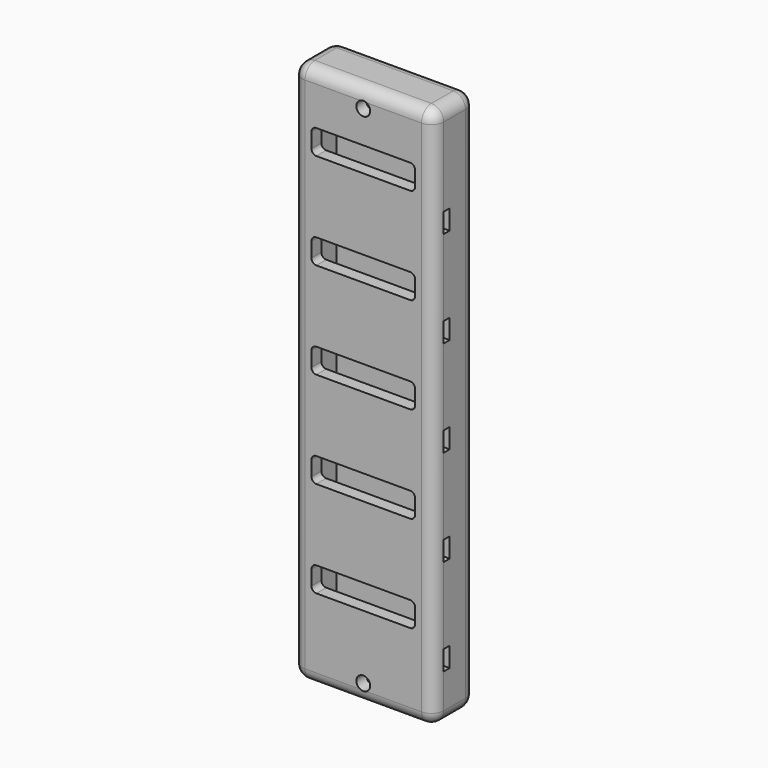
from build123d import *

# Parameters (mm, degrees)
F0_W         = 29.972
F0_H         = 5.08
F0_H_2       = 2.54
F0_R         = 1.7145
F0_H_3       = 13.97
F0_W_2       = 3.175
F1_DEPTH     = 10.16
F2_DEPTH     = 6.985
F3_DEPTH     = 1.905
F4_T1_DEPTH  = 133.35
F4_T3_DEPTH  = 14.9225
F4_T5_DEPTH  = 29.972
F4_S9_W      = 3.175
F4_S9_H      = 3.175
F4_T10_DEPTH = 3.175
F4_S15_W     = 3.175
F4_S15_H     = 3.175
F4_T16_DEPTH = 3.175
F4_S21_W     = 3.175
F4_S21_H     = 3.175
F4_T22_DEPTH = 3.175
F4_S27_W     = 3.175
F4_S27_H     = 3.175
F4_T28_DEPTH = 3.175
F5_R         = 1.778
F6_DEPTH     = 3.175
F7_T1_DEPTH  = 133.35
F7_T3_DEPTH  = 29.972
F7_T6_ANGLE  = 90
F7_T8_ANGLE  = 90
F7_T10_ANGLE = 90
F7_T12_ANGLE = 90


# Not quite as in the source:
# - a fillet or chamfer that OpenCascade refuses, or shapes differently, is made with other operations: its cross-section is extruded or revolved along the edge and cut away or added


with BuildPart() as f1:
    # F0 (on Front) → F1 (new body)
    with BuildSketch(Plane.XZ):
        with Locations((0, 14.605)):
            Rectangle(F0_W, F0_H)
        Polygon((-18.161, 86.36), (-18.161, 66.675), (-14.986, 66.675), (-14.986, 80.645), (14.986, 80.645), (14.986, 66.675), (18.161, 66.675), (18.161, 86.36), (14.986, 86.36), (14.986, 83.82), (-14.986, 83.82), (-14.986, 86.36), align=None)
        with Locations((0, 60.325)):
            Rectangle(F0_W, F0_H_2)
        Polygon((-18.161, 12.065), (-18.161, 0), (18.161, 0), (18.161, 12.065), (14.986, 12.065), (14.986, 9.525), (-14.986, 9.525), (-14.986, 12.065), align=None)
        with Locations((0, 4.7625)):
            Circle(F0_R, mode=Mode.SUBTRACT)
        with Locations((0, 85.09)):
            Rectangle(F0_W, F0_H_2)
        with Locations((0, 98.425)):
            Rectangle(F0_W, F0_H_3)
        Polygon((-18.161, 139.7), (-18.161, 116.205), (-14.986, 116.205), (-14.986, 130.175), (14.986, 130.175), (14.986, 116.205), (18.161, 116.205), (18.161, 139.7), align=None)
        with Locations((0, 134.9375)):
            Circle(F0_R, mode=Mode.SUBTRACT)
        with Locations((0, 48.895)):
            Rectangle(F0_W, F0_H_3)
        with Locations((0, 10.795)):
            Rectangle(F0_W, F0_H_2)
        with Locations((-16.5735, 39.37)):
            Rectangle(F0_W_2, F0_H)
        with Locations((0, 73.66)):
            Rectangle(F0_W, F0_H_3)
        with Locations((-16.5735, 14.605)):
            Rectangle(F0_W_2, F0_H)
        with Locations((0, 123.19)):
            Rectangle(F0_W, F0_H_3)
        with Locations((0, 109.855)):
            Rectangle(F0_W, F0_H_2)
        with Locations((0, 24.13)):
            Rectangle(F0_W, F0_H_3)
        with Locations((0, 35.56)):
            Rectangle(F0_W, F0_H_2)
        with Locations((-16.5735, 113.665)):
            Rectangle(F0_W_2, F0_H)
        with Locations((-16.5735, 64.135)):
            Rectangle(F0_W_2, F0_H)
        with Locations((0, 113.665)):
            Rectangle(F0_W, F0_H)
        Polygon((-18.161, 36.83), (-18.161, 17.145), (-14.986, 17.145), (-14.986, 31.115), (14.986, 31.115), (14.986, 17.145), (18.161, 17.145), (18.161, 36.83), (14.986, 36.83), (14.986, 34.29), (-14.986, 34.29), (-14.986, 36.83), align=None)
        with Locations((0, 39.37)):
            Rectangle(F0_W, F0_H)
        Polygon((-18.161, 111.125), (-18.161, 91.44), (-14.986, 91.44), (-14.986, 105.41), (14.986, 105.41), (14.986, 91.44), (18.161, 91.44), (18.161, 111.125), (14.986, 111.125), (14.986, 108.585), (-14.986, 108.585), (-14.986, 111.125), align=None)
        Polygon((-18.161, 61.595), (-18.161, 41.91), (-14.986, 41.91), (-14.986, 55.88), (14.986, 55.88), (14.986, 41.91), (18.161, 41.91), (18.161, 61.595), (14.986, 61.595), (14.986, 59.055), (-14.986, 59.055), (-14.986, 61.595), align=None)
        with Locations((0, 64.135)):
            Rectangle(F0_W, F0_H)
        with Locations((-16.5735, 88.9)):
            Rectangle(F0_W_2, F0_H)
        with Locations((0, 88.9)):
            Rectangle(F0_W, F0_H)
        with Locations((16.5735, 39.37)):
            Rectangle(F0_W_2, F0_H)
        with Locations((16.5735, 14.605)):
            Rectangle(F0_W_2, F0_H)
        with Locations((16.5735, 88.9)):
            Rectangle(F0_W_2, F0_H)
        with Locations((16.5735, 113.665)):
            Rectangle(F0_W_2, F0_H)
        with Locations((16.5735, 64.135)):
            Rectangle(F0_W_2, F0_H)
    extrude(amount=-F1_DEPTH)

    # F0 (on Front) → F2 (cut)
    with BuildSketch(Plane.XZ):
        with Locations((0, 98.425)):
            Rectangle(F0_W, F0_H_3)
        with Locations((0, 35.56)):
            Rectangle(F0_W, F0_H_2)
        with Locations((0, 48.895)):
            Rectangle(F0_W, F0_H_3)
        with Locations((0, 64.135)):
            Rectangle(F0_W, F0_H)
        with Locations((0, 14.605)):
            Rectangle(F0_W, F0_H)
        with Locations((0, 10.795)):
            Rectangle(F0_W, F0_H_2)
        with Locations((0, 113.665)):
            Rectangle(F0_W, F0_H)
        with Locations((0, 88.9)):
            Rectangle(F0_W, F0_H)
        with Locations((0, 123.19)):
            Rectangle(F0_W, F0_H_3)
        with Locations((0, 60.325)):
            Rectangle(F0_W, F0_H_2)
        with Locations((0, 24.13)):
            Rectangle(F0_W, F0_H_3)
        with Locations((0, 73.66)):
            Rectangle(F0_W, F0_H_3)
        with Locations((0, 39.37)):
            Rectangle(F0_W, F0_H)
        with Locations((0, 85.09)):
            Rectangle(F0_W, F0_H_2)
        with Locations((0, 109.855)):
            Rectangle(F0_W, F0_H_2)
    extrude(amount=-F2_DEPTH, mode=Mode.SUBTRACT)

    # F0 (on Front) → F3 (cut)
    with BuildSketch(Plane.XZ):
        with Locations((-16.5735, 14.605)):
            Rectangle(F0_W_2, F0_H)
        with Locations((0, 14.605)):
            Rectangle(F0_W, F0_H)
        with Locations((16.5735, 14.605)):
            Rectangle(F0_W_2, F0_H)
        with Locations((16.5735, 39.37)):
            Rectangle(F0_W_2, F0_H)
        with Locations((0, 39.37)):
            Rectangle(F0_W, F0_H)
        with Locations((-16.5735, 39.37)):
            Rectangle(F0_W_2, F0_H)
        with Locations((-16.5735, 88.9)):
            Rectangle(F0_W_2, F0_H)
        with Locations((0, 88.9)):
            Rectangle(F0_W, F0_H)
        with Locations((16.5735, 88.9)):
            Rectangle(F0_W_2, F0_H)
        with Locations((16.5735, 64.135)):
            Rectangle(F0_W_2, F0_H)
        with Locations((0, 64.135)):
            Rectangle(F0_W, F0_H)
        with Locations((-16.5735, 64.135)):
            Rectangle(F0_W_2, F0_H)
        with Locations((-16.5735, 113.665)):
            Rectangle(F0_W_2, F0_H)
        with Locations((0, 113.665)):
            Rectangle(F0_W, F0_H)
        with Locations((16.5735, 113.665)):
            Rectangle(F0_W_2, F0_H)
    extrude(amount=-F3_DEPTH, mode=Mode.SUBTRACT)

    # F4: fillet of radius 3.175 on 8 edges, made by hand

    # F4_s2 → F4_t1 (cut)
    with BuildSketch(Plane.XY.offset(3.175)):
        with BuildLine():
            ThreePointArc((18.161, 6.985), (17.2310640303, 9.2300640303), (14.986, 10.16))
            Line((14.986, 10.16), (18.161, 10.16))
            Line((18.161, 10.16), (18.161, 6.985))
        make_face()
        with BuildLine():
            ThreePointArc((-18.161, 6.985), (-17.2310640303, 9.2300640303), (-14.986, 10.16))
            Line((-14.986, 10.16), (-18.161, 10.16))
            Line((-18.161, 10.16), (-18.161, 6.985))
        make_face()
    extrude(amount=F4_T1_DEPTH, mode=Mode.SUBTRACT)

    # F4_s4 → F4_t3 (cut)
    with BuildSketch(Plane.XZ.offset(-6.985)):
        with BuildLine():
            ThreePointArc((18.161, 136.525), (17.2310640303, 138.7700640303), (14.986, 139.7))
            Line((14.986, 139.7), (18.161, 139.7))
            Line((18.161, 139.7), (18.161, 136.525))
        make_face()
        with BuildLine():
            ThreePointArc((-18.161, 136.525), (-17.2310640303, 138.7700640303), (-14.986, 139.7))
            Line((-14.986, 139.7), (-18.161, 139.7))
            Line((-18.161, 139.7), (-18.161, 136.525))
        make_face()
        with BuildLine():
            ThreePointArc((-14.986, 0), (-17.2310640303, 0.9299359697), (-18.161, 3.175))
            Line((-18.161, 3.175), (-18.161, 0))
            Line((-18.161, 0), (-14.986, 0))
        make_face()
        with BuildLine():
            ThreePointArc((14.986, 0), (17.2310640303, 0.9299359697), (18.161, 3.175))
            Line((18.161, 3.175), (18.161, 0))
            Line((18.161, 0), (14.986, 0))
        make_face()
    extrude(amount=F4_T3_DEPTH, mode=Mode.SUBTRACT)

    # F4_s6 → F4_t5 (cut)
    with BuildSketch(Plane.YZ.offset(-14.986)):
        with BuildLine():
            ThreePointArc((6.985, 0), (9.2300640303, 0.9299359697), (10.16, 3.175))
            Line((10.16, 3.175), (10.16, 0))
            Line((10.16, 0), (6.985, 0))
        make_face()
        with BuildLine():
            ThreePointArc((10.16, 136.525), (9.2300640303, 138.7700640303), (6.985, 139.7))
            Line((6.985, 139.7), (10.16, 139.7))
            Line((10.16, 139.7), (10.16, 136.525))
        make_face()
    extrude(amount=F4_T5_DEPTH, mode=Mode.SUBTRACT)


with BuildPart() as f4_tool8:
    # F4_s9 → F4_t10 (new body)
    with BuildSketch(Plane.XY.offset(3.175)):
        with Locations((16.5735, 8.5725)):
            Rectangle(F4_S9_W, F4_S9_H)
    extrude(amount=-F4_T10_DEPTH)

    # F4_s11 → F4_t12 (revolve, cut)
    with BuildSketch(Plane(origin=(14.986, 6.985, 3.175), x_dir=(-0.7071067812, -0.7071067812, 0), z_dir=(0.7071067812, -0.7071067812, 0))):
        with BuildLine():
            ThreePointArc((0, -3.175), (3.175, 0), (0, 3.175))
            Line((0, 3.175), (0, -3.175))
        make_face()
    revolve(axis=Axis((14.986, 6.985, 3.175), (0, 0, -1)), mode=Mode.SUBTRACT)


with BuildPart() as f1_1:
    add(f1.part)

    # F4_t7: cut F4_tool8
    add(f4_tool8.part, mode=Mode.SUBTRACT)


with BuildPart() as f4_tool14:
    # F4_s15 → F4_t16 (new body)
    with BuildSketch(Plane.XY.offset(136.525)):
        with Locations((16.5735, 8.5725)):
            Rectangle(F4_S15_W, F4_S15_H)
    extrude(amount=F4_T16_DEPTH)

    # F4_s17 → F4_t18 (revolve, cut)
    with BuildSketch(Plane(origin=(14.986, 6.985, 136.525), x_dir=(-0.7071067812, -0.7071067812, 0), z_dir=(-0.7071067812, 0.7071067812, 0))):
        with BuildLine():
            ThreePointArc((0, -3.175), (3.175, 0), (0, 3.175))
            Line((0, 3.175), (0, -3.175))
        make_face()
    revolve(axis=Axis((14.986, 6.985, 136.525), (0, 0, 1)), mode=Mode.SUBTRACT)


with BuildPart() as f1_2:
    add(f1_1.part)

    # F4_t13: cut F4_tool14
    add(f4_tool14.part, mode=Mode.SUBTRACT)


with BuildPart() as f4_tool20:
    # F4_s21 → F4_t22 (new body)
    with BuildSketch(Plane.YZ.offset(-14.986)):
        with Locations((8.5725, 138.1125)):
            Rectangle(F4_S21_W, F4_S21_H)
    extrude(amount=-F4_T22_DEPTH)

    # F4_s23 → F4_t24 (revolve, cut)
    with BuildSketch(Plane(origin=(-14.986, 6.985, 136.525), x_dir=(0, -0.7071067812, -0.7071067812), z_dir=(0, 0.7071067812, -0.7071067812))):
        with BuildLine():
            ThreePointArc((0, -3.175), (3.175, 0), (0, 3.175))
            Line((0, 3.175), (0, -3.175))
        make_face()
    revolve(axis=Axis((-14.986, 6.985, 136.525), (-1, 0, 0)), mode=Mode.SUBTRACT)


with BuildPart() as f1_3:
    add(f1_2.part)

    # F4_t19: cut F4_tool20
    add(f4_tool20.part, mode=Mode.SUBTRACT)


with BuildPart() as f4_tool26:
    # F4_s27 → F4_t28 (new body)
    with BuildSketch(Plane.XY.offset(3.175)):
        with Locations((-16.5735, 8.5725)):
            Rectangle(F4_S27_W, F4_S27_H)
    extrude(amount=-F4_T28_DEPTH)

    # F4_s29 → F4_t30 (revolve, cut)
    with BuildSketch(Plane(origin=(-14.986, 6.985, 3.175), x_dir=(0.7071067812, -0.7071067812, 0), z_dir=(0.7071067812, 0.7071067812, 0))):
        with BuildLine():
            ThreePointArc((0, -3.175), (3.175, 0), (0, 3.175))
            Line((0, 3.175), (0, -3.175))
        make_face()
    revolve(axis=Axis((-14.986, 6.985, 3.175), (0, 0, -1)), mode=Mode.SUBTRACT)


with BuildPart() as f1_4:
    add(f1_3.part)

    # F4_t25: cut F4_tool26
    add(f4_tool26.part, mode=Mode.SUBTRACT)


with BuildPart() as f6:
    # F5 (on Front) → F6 (new body)
    with BuildSketch(Plane.XZ):
        with BuildLine():
            ThreePointArc((-18.161, 3.175), (-17.2310640303, 0.9299359697), (-14.986, 0))
            Line((-14.986, 0), (14.986, 0))
            ThreePointArc((14.986, 0), (17.2310640303, 0.9299359697), (18.161, 3.175))
            Line((18.161, 3.175), (18.161, 136.525))
            ThreePointArc((18.161, 136.525), (17.2310640303, 138.7700640303), (14.986, 139.7))
            Line((14.986, 139.7), (-14.986, 139.7))
            ThreePointArc((-14.986, 139.7), (-17.2310640303, 138.7700640303), (-18.161, 136.525))
            Line((-18.161, 136.525), (-18.161, 3.175))
        make_face()
        with Locations((0, 4.7625)):
            Circle(F5_R, mode=Mode.SUBTRACT)
        with BuildLine():
            Line((12.065, 21.209), (-12.065, 21.209))
            ThreePointArc((-12.065, 21.209), (-12.9630256121, 21.5809743879), (-13.335, 22.479))
            Line((-13.335, 22.479), (-13.335, 26.289))
            ThreePointArc((-13.335, 26.289), (-12.9630256121, 27.1870256121), (-12.065, 27.559))
            Line((-12.065, 27.559), (12.065, 27.559))
            ThreePointArc((12.065, 27.559), (12.9630256121, 27.1870256121), (13.335, 26.289))
            Line((13.335, 26.289), (13.335, 22.479))
            ThreePointArc((13.335, 22.479), (12.9630256121, 21.5809743879), (12.065, 21.209))
        make_face(mode=Mode.SUBTRACT)
        with BuildLine():
            Line((12.065, 45.974), (-12.065, 45.974))
            ThreePointArc((-12.065, 45.974), (-12.9630256121, 46.3459743879), (-13.335, 47.244))
            Line((-13.335, 47.244), (-13.335, 51.054))
            ThreePointArc((-13.335, 51.054), (-12.9630256121, 51.9520256121), (-12.065, 52.324))
            Line((-12.065, 52.324), (12.065, 52.324))
            ThreePointArc((12.065, 52.324), (12.9630256121, 51.9520256121), (13.335, 51.054))
            Line((13.335, 51.054), (13.335, 47.244))
            ThreePointArc((13.335, 47.244), (12.9630256121, 46.3459743879), (12.065, 45.974))
        make_face(mode=Mode.SUBTRACT)
        with BuildLine():
            Line((12.065, 70.739), (-12.065, 70.739))
            ThreePointArc((-12.065, 70.739), (-12.9630256121, 71.1109743879), (-13.335, 72.009))
            Line((-13.335, 72.009), (-13.335, 75.819))
            ThreePointArc((-13.335, 75.819), (-12.9630256121, 76.7170256121), (-12.065, 77.089))
            Line((-12.065, 77.089), (12.065, 77.089))
            ThreePointArc((12.065, 77.089), (12.9630256121, 76.7170256121), (13.335, 75.819))
            Line((13.335, 75.819), (13.335, 72.009))
            ThreePointArc((13.335, 72.009), (12.9630256121, 71.1109743879), (12.065, 70.739))
        make_face(mode=Mode.SUBTRACT)
        with BuildLine():
            Line((12.065, 95.504), (-12.065, 95.504))
            ThreePointArc((-12.065, 95.504), (-12.9630256121, 95.8759743879), (-13.335, 96.774))
            Line((-13.335, 96.774), (-13.335, 100.584))
            ThreePointArc((-13.335, 100.584), (-12.9630256121, 101.4820256121), (-12.065, 101.854))
            Line((-12.065, 101.854), (12.065, 101.854))
            ThreePointArc((12.065, 101.854), (12.9630256121, 101.4820256121), (13.335, 100.584))
            Line((13.335, 100.584), (13.335, 96.774))
            ThreePointArc((13.335, 96.774), (12.9630256121, 95.8759743879), (12.065, 95.504))
        make_face(mode=Mode.SUBTRACT)
        with BuildLine():
            Line((12.065, 120.269), (-12.065, 120.269))
            ThreePointArc((-12.065, 120.269), (-12.9630256121, 120.6409743879), (-13.335, 121.539))
            Line((-13.335, 121.539), (-13.335, 125.349))
            ThreePointArc((-13.335, 125.349), (-12.9630256121, 126.2470256121), (-12.065, 126.619))
            Line((-12.065, 126.619), (12.065, 126.619))
            ThreePointArc((12.065, 126.619), (12.9630256121, 126.2470256121), (13.335, 125.349))
            Line((13.335, 125.349), (13.335, 121.539))
            ThreePointArc((13.335, 121.539), (12.9630256121, 120.6409743879), (12.065, 120.269))
        make_face(mode=Mode.SUBTRACT)
        with Locations((0, 134.9375)):
            Circle(F5_R, mode=Mode.SUBTRACT)
    extrude(amount=F6_DEPTH)

    # F7: fillet of radius 3.175 on 8 edges, made by hand

    # F7_s2 → F7_t1 (cut)
    with BuildSketch(Plane.XY.offset(3.175)):
        with BuildLine():
            ThreePointArc((18.161, 0), (17.2310640303, -2.2450640303), (14.986, -3.175))
            Line((14.986, -3.175), (18.161, -3.175))
            Line((18.161, -3.175), (18.161, 0))
        make_face()
        with BuildLine():
            ThreePointArc((-18.161, 0), (-17.2310640303, -2.2450640303), (-14.986, -3.175))
            Line((-14.986, -3.175), (-18.161, -3.175))
            Line((-18.161, -3.175), (-18.161, 0))
        make_face()
    extrude(amount=F7_T1_DEPTH, mode=Mode.SUBTRACT)

    # F7_s4 → F7_t3 (cut)
    with BuildSketch(Plane.YZ.offset(-14.986)):
        with BuildLine():
            ThreePointArc((0, 0), (-2.2450640303, 0.9299359697), (-3.175, 3.175))
            Line((-3.175, 3.175), (-3.175, 0))
            Line((-3.175, 0), (0, 0))
        make_face()
        with BuildLine():
            ThreePointArc((0, 139.7), (-2.2450640303, 138.7700640303), (-3.175, 136.525))
            Line((-3.175, 136.525), (-3.175, 139.7))
            Line((-3.175, 139.7), (0, 139.7))
        make_face()
    extrude(amount=F7_T3_DEPTH, mode=Mode.SUBTRACT)

    # F7_s5 → F7_t6 (revolve, cut)
    with BuildSketch(Plane.XY.offset(3.175)):
        with BuildLine():
            ThreePointArc((-18.161, 0), (-17.2310640303, -2.2450640303), (-14.986, -3.175))
            Line((-14.986, -3.175), (-18.161, -3.175))
            Line((-18.161, -3.175), (-18.161, 0))
        make_face()
    revolve(axis=Axis((-14.986, -3.175, 3.175), (0, -1, 0)), revolution_arc=F7_T6_ANGLE, mode=Mode.SUBTRACT)

    # F7_s7 → F7_t8 (revolve, cut)
    with BuildSketch(Plane.YZ.offset(14.986)):
        with BuildLine():
            ThreePointArc((0, 0), (-2.2450640303, 0.9299359697), (-3.175, 3.175))
            Line((-3.175, 3.175), (-3.175, 0))
            Line((-3.175, 0), (0, 0))
        make_face()
    revolve(axis=Axis((14.986, -3.175, 3.175), (0, -1, 0)), revolution_arc=F7_T8_ANGLE, mode=Mode.SUBTRACT)

    # F7_s9 → F7_t10 (revolve, cut)
    with BuildSketch(Plane.XY.offset(136.525)):
        with BuildLine():
            ThreePointArc((18.161, 0), (17.2310640303, -2.2450640303), (14.986, -3.175))
            Line((14.986, -3.175), (18.161, -3.175))
            Line((18.161, -3.175), (18.161, 0))
        make_face()
    revolve(axis=Axis((14.986, -3.175, 136.525), (0, -1, 0)), revolution_arc=F7_T10_ANGLE, mode=Mode.SUBTRACT)

    # F7_s11 → F7_t12 (revolve, cut)
    with BuildSketch(Plane.YZ.offset(-14.986)):
        with BuildLine():
            ThreePointArc((0, 139.7), (-2.2450640303, 138.7700640303), (-3.175, 136.525))
            Line((-3.175, 136.525), (-3.175, 139.7))
            Line((-3.175, 139.7), (0, 139.7))
        make_face()
    revolve(axis=Axis((-14.986, -3.175, 136.525), (0, -1, 0)), revolution_arc=F7_T12_ANGLE, mode=Mode.SUBTRACT)


solid = Compound([f1_4.part, f6.part])
